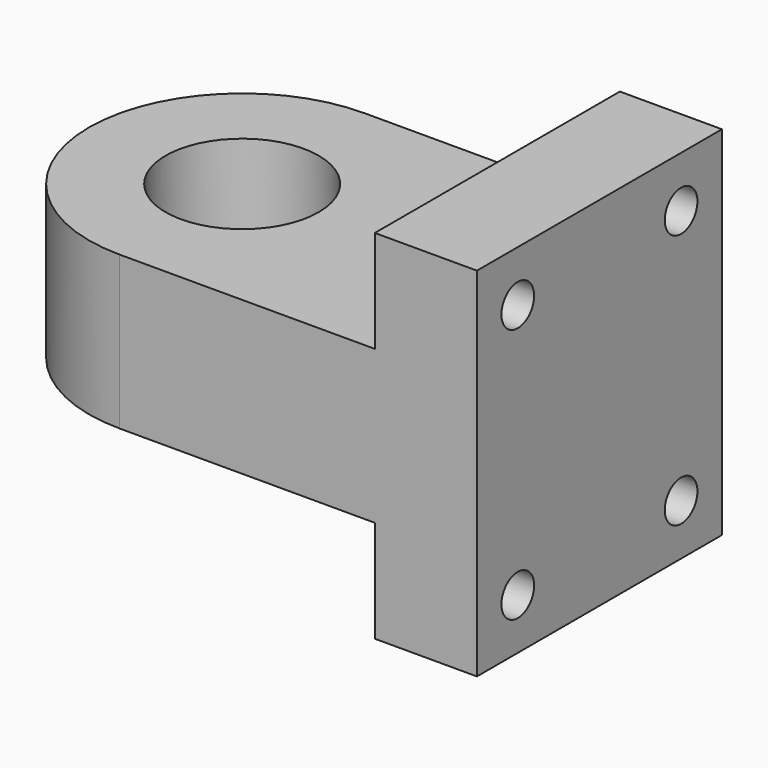
from build123d import *

# Parameters (mm, degrees)
F1_DEPTH = 30
F2_R     = 30
F3_R     = 29.99999
F4_R     = 15
F5_DEPTH = 15
F7_R     = 4
F8_DEPTH = 20


# Not quite as in the source:
# - a fillet or chamfer is up to 0.001 mm smaller than in the source, because OpenCascade refuses the exact size


with BuildPart() as f1:
    # F0 (on Front) → F1 (new body, symmetric)
    with BuildSketch(Plane.XZ):
        Polygon((-100, 0), (0, 0), (0, 35), (-20, 35), (-20, 15), (-100, 15), align=None)
    extrude(amount=F1_DEPTH, both=True)

    # F2
    f2_edges = [f1.edges().sort_by_distance(p)[0] for p in [
        (-100, -30, 7.5),
    ]]
    fillet(f2_edges, radius=F2_R)

    # F3 (radius 30 in the source; OpenCascade refuses exactly that, so slightly less here)
    f3_edges = [f1.edges().sort_by_distance(p)[0] for p in [
        (-100, 30, 7.5),
    ]]
    fillet(f3_edges, radius=F3_R)

    # F4 (on face) → F5 (cut, through all)
    with BuildSketch(Plane.XY.offset(15)):
        with Locations((-70, 0)):
            Circle(F4_R)
    extrude(amount=-F5_DEPTH, mode=Mode.SUBTRACT)

    # F6: F1 across plane


with BuildPart() as f1_1:
    add(f1.part)
    add(f1.part.mirror(Plane.XY))

    # F7 (on face) → F8 (cut, through all)
    with BuildSketch(Plane.YZ):
        with BuildLine():
            ThreePointArc((-24, -25), (-20, -29), (-16, -25))
            ThreePointArc((-16, -25), (-20, -21), (-24, -25))
        make_face()
        with Locations((-20, 25)):
            Circle(F7_R)
        with Locations((20, -25)):
            Circle(F7_R)
        with Locations((20, 25)):
            Circle(F7_R)
    extrude(amount=-F8_DEPTH, mode=Mode.SUBTRACT)


solid = f1_1.part
